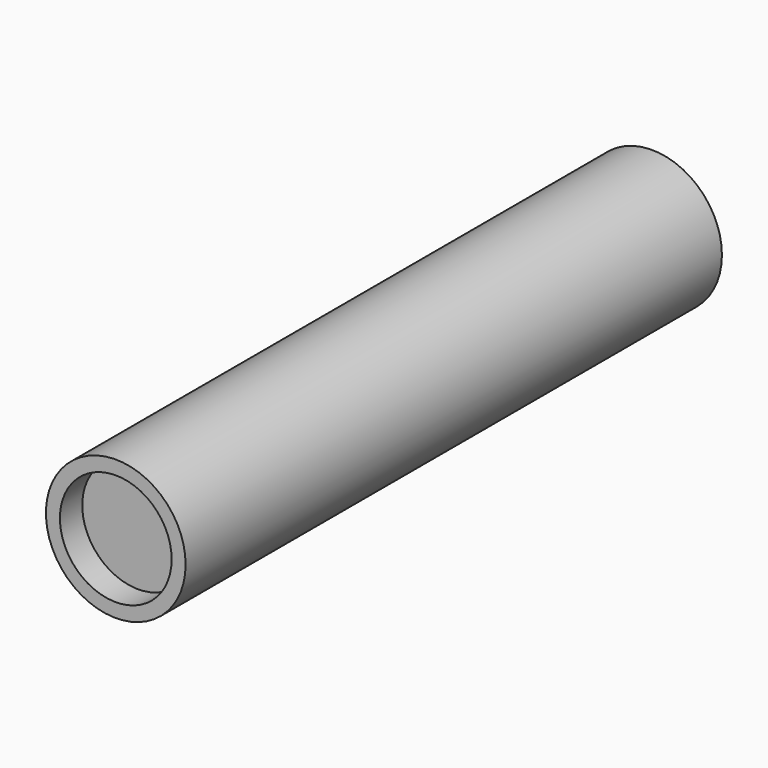
from build123d import *

# Parameters (mm, degrees)
F0_R      = 31.75
F0_R_2    = 25.4
F1_DEPTH  = 304.8
F0_R_3    = 12.7
F2_DEPTH  = 76.2
F0_R_4    = 9.525
F4_DEPTH  = 76.2
F6_SIZE2  = 11.7317574699
F6_SIZE   = 20.32
F7_SIZE2  = 11.5700461292
F7_SIZE   = 43.18
F8_R      = 19.05
F9_R      = 44.45
F10_SIZE2 = 14.81177
F10_SIZE  = 76.19999
F13_DEPTH = 19.05


# Not quite as in the source:
# - a fillet or chamfer is up to 0.001 mm smaller than in the source, because OpenCascade refuses the exact size


with BuildPart() as f1:
    # F0 (on Front) → F1 (new body)
    with BuildSketch(Plane.XZ):
        Circle(F0_R)
        Circle(F0_R_2, mode=Mode.SUBTRACT)
    extrude(amount=-F1_DEPTH)


with BuildPart() as f2:
    # F0 (on Front) → F2 (new body)
    with BuildSketch(Plane.XZ):
        Circle(F0_R_2)
        Circle(F0_R_3, mode=Mode.SUBTRACT)
    extrude(amount=-F2_DEPTH)


with BuildPart() as f2_1:
    # F3: moved
    add(f2.part.moved(Location((127, 0, 0))))

    # F6
    f6_edges = [f2_1.edges().sort_by_distance(p)[0] for p in [
        (114.3, 0, 0),
    ]]
    chamfer(f6_edges, length=F6_SIZE, length2=F6_SIZE2)

    # F7
    f7_edges = [f2_1.edges().sort_by_distance(p)[0] for p in [
        (114.3, 76.2, 0),
    ]]
    chamfer(f7_edges, length=F7_SIZE, length2=F7_SIZE2)

    # F8
    f8_edges = [f2_1.edges().sort_by_distance(p)[0] for p in [
        (114.3, 20.32, 0),
    ]]
    fillet(f8_edges, radius=F8_R)

    # F9
    f9_edges = [f2_1.edges().sort_by_distance(p)[0] for p in [
        (114.3, 33.02, 0),
    ]]
    fillet(f9_edges, radius=F9_R)


with BuildPart() as f4:
    # F0 (on Front) → F4 (new body)
    with BuildSketch(Plane.XZ):
        Circle(F0_R_2)
        Circle(F0_R_3, mode=Mode.SUBTRACT)
        Circle(F0_R_3)
        Circle(F0_R_4, mode=Mode.SUBTRACT)
    extrude(amount=-F4_DEPTH)


with BuildPart() as f4_1:
    # F5: moved
    add(f4.part.moved(Location((-127, 0, 0))))

    # F10 (size 76.2 and 14.8117795563 in the source; OpenCascade refuses exactly that, so slightly less here)
    f10_edges = [f4_1.edges().sort_by_distance(p)[0] for p in [
        (-136.525, 0, 0),
    ]]
    f10_side = f4_1.faces().sort_by_distance((-136.525, 38.1, 0))[0]
    chamfer(f10_edges, length=F10_SIZE, length2=F10_SIZE2, reference=f10_side)


with BuildPart() as f4_2:
    # F11: moved
    add(f4_1.part.moved(Location((127, 228.6, 0))))


with BuildPart() as f2_2:
    # F12: moved
    add(f2_1.part.moved(Location((-127, 139.7, 0))))


with BuildPart() as f13:
    # F0 (on Front) → F13 (new body)
    with BuildSketch(Plane.XZ):
        Circle(F0_R_2)
        Circle(F0_R_3, mode=Mode.SUBTRACT)
        Circle(F0_R_3)
        Circle(F0_R_4, mode=Mode.SUBTRACT)
        Circle(F0_R_4)
    extrude(amount=-F13_DEPTH)


with BuildPart() as f13_1:
    # F14: moved
    add(f13.part.moved(Location((0, 12.7, 0))))


solid = Compound([f1.part, f4_2.part, f2_2.part, f13_1.part])
